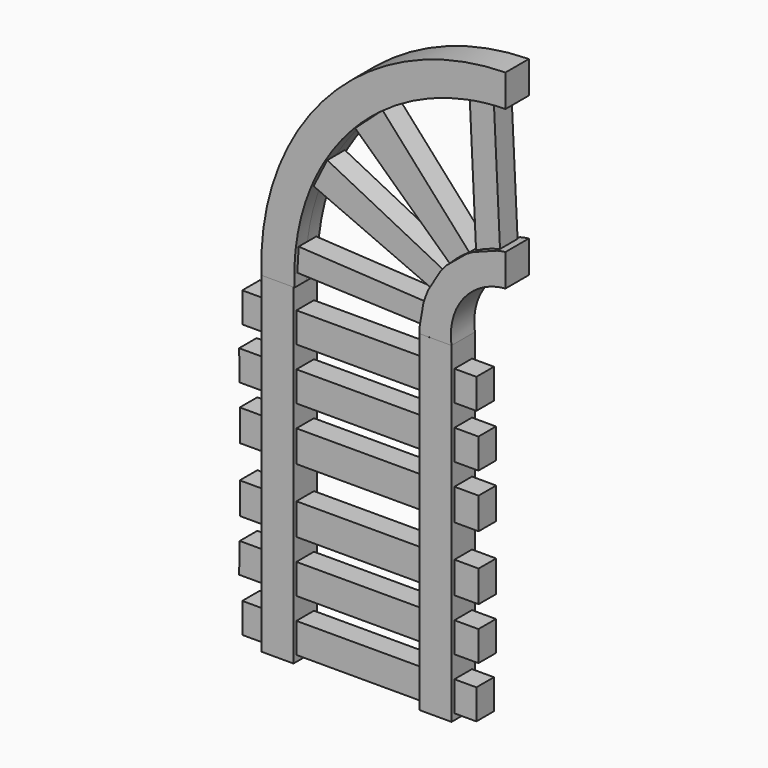
from build123d import *

# Parameters (mm, degrees)
F0_W          = 11.176
F0_H          = 7.62
F0_H_2        = 10.414
F0_H_3        = 10.414198041
F0_H_4        = 10.8981402591
F0_H_5        = 11.3893379234
F0_H_6        = 2.1167141254
F1_DEPTH      = 5.08
F1_DEPTH_BACK = 5.08
F0_W_2        = 43.688
F0_W_3        = 7.62
F0_W_4        = 8.491490941
F0_W_5        = 8.3875925946
F0_W_6        = 8.3293178785
F2_DEPTH      = 3.81
F2_DEPTH_BACK = 3.81
F4_DEPTH      = 5.08
F4_DEPTH_BACK = 5.08
F5_DEPTH      = 3.81
F5_DEPTH_BACK = 3.81


# Not quite as in the source:
# - a feature names something its author has since deleted; it is built from what else it names


with BuildPart() as f1:
    # F0 (on Front) → F1 (new body, two sides)
    with BuildSketch(Plane.XZ) as f1_sk:
        with Locations((-27.432, 56.4710072617)):
            Rectangle(F0_W, F0_H)
        with Locations((-27.432, 47.4540072617)):
            Rectangle(F0_W, F0_H_2)
        with Locations((-27.432, 38.4370072617)):
            Rectangle(F0_W, F0_H)
        with Locations((-27.432, 29.4199082413)):
            Rectangle(F0_W, F0_H_3)
        with Locations((-27.432, 20.4028092208)):
            Rectangle(F0_W, F0_H)
        with Locations((-27.432, 11.1437390912)):
            Rectangle(F0_W, F0_H_4)
        with Locations((-27.432, 0)):
            Rectangle(F0_W, F0_H_5)
        with Locations((-27.432, -11.1437390912)):
            Rectangle(F0_W, F0_H_4)
        with Locations((-27.432, -20.4028092208)):
            Rectangle(F0_W, F0_H)
        with Locations((-27.432, -29.4199082413)):
            Rectangle(F0_W, F0_H_3)
        with Locations((-27.432, -38.4370072617)):
            Rectangle(F0_W, F0_H)
        with Locations((-27.432, -47.4540072617)):
            Rectangle(F0_W, F0_H_2)
        with Locations((-27.432, -53.7193643245)):
            Rectangle(F0_W, F0_H_6)
    extrude(amount=F1_DEPTH)
    extrude(f1_sk.sketch, amount=-F1_DEPTH_BACK)



with BuildPart() as f1b:
    # F0 (on Front) → F1, piece 2 (new body, two sides)
    with BuildSketch(Plane.XZ) as f1_2_sk:
        with Locations((27.432, -47.4540072617)):
            Rectangle(F0_W, F0_H_2)
        with Locations((27.432, -38.4370072617)):
            Rectangle(F0_W, F0_H)
        with Locations((27.432, -29.4199082413)):
            Rectangle(F0_W, F0_H_3)
        with Locations((27.432, -20.4028092208)):
            Rectangle(F0_W, F0_H)
        with Locations((27.432, -11.1437390912)):
            Rectangle(F0_W, F0_H_4)
        with Locations((27.432, 0)):
            Rectangle(F0_W, F0_H_5)
        with Locations((27.432, 11.1437390912)):
            Rectangle(F0_W, F0_H_4)
        with Locations((27.432, 20.4028092208)):
            Rectangle(F0_W, F0_H)
        with Locations((27.432, 29.4199082413)):
            Rectangle(F0_W, F0_H_3)
        with Locations((27.432, 38.4370072617)):
            Rectangle(F0_W, F0_H)
        with Locations((27.432, 47.4540072617)):
            Rectangle(F0_W, F0_H_2)
        with Locations((27.432, 56.4710072617)):
            Rectangle(F0_W, F0_H)
        with Locations((27.432, -53.7193643245)):
            Rectangle(F0_W, F0_H_6)
    extrude(amount=F1_DEPTH)
    extrude(f1_2_sk.sketch, amount=-F1_DEPTH_BACK)


with BuildPart() as f1_1:
    add(f1.part)

    add(f1b.part)  # F2 merges F1b
    # F0 (on Front) → F2 (join, two sides)
    with BuildSketch(Plane.XZ) as f2_sk:
        with Locations((0, 29.4199082413)):
            Rectangle(F0_W_2, F0_H_3)
        with Locations((0, 47.4540072617)):
            Rectangle(F0_W_2, F0_H_2)
        with Locations((-36.83, 47.4540072617)):
            Rectangle(F0_W_3, F0_H_2)
        Polygon((-33.02, 24.2128092208), (-33.02, 34.6270072617), (-41.7378880084, 34.6270072617), (-41.511490941, 24.2128092208), align=None)
        with Locations((-37.2657454705, 11.1437390912)):
            Rectangle(F0_W_4, F0_H_4)
        with Locations((-37.2657454705, -11.1437390912)):
            Rectangle(F0_W_4, F0_H_4)
        with Locations((0, -11.1437390912)):
            Rectangle(F0_W_2, F0_H_4)
        with Locations((0, 11.1437390912)):
            Rectangle(F0_W_2, F0_H_4)
        with Locations((37.2137962973, -11.1437390912)):
            Rectangle(F0_W_5, F0_H_4)
        with Locations((37.2137962973, 11.1437390912)):
            Rectangle(F0_W_5, F0_H_4)
        with Locations((37.1846589392, 29.4199082413)):
            Rectangle(F0_W_6, F0_H_3)
        with Locations((36.83, 47.4540072617)):
            Rectangle(F0_W_3, F0_H_2)
        with Locations((37.1846589392, -29.4199082413)):
            Rectangle(F0_W_6, F0_H_3)
        with Locations((36.83, -47.4540072617)):
            Rectangle(F0_W_3, F0_H_2)
        with Locations((0, -47.4540072617)):
            Rectangle(F0_W_2, F0_H_2)
        with Locations((0, -29.4199082413)):
            Rectangle(F0_W_2, F0_H_3)
        Polygon((-33.02, -34.6270072617), (-33.02, -24.2128092208), (-41.511490941, -24.2128092208), (-41.7378880084, -34.6270072617), align=None)
        with Locations((-36.83, -47.4540072617)):
            Rectangle(F0_W_3, F0_H_2)
    extrude(amount=F2_DEPTH)
    extrude(f2_sk.sketch, amount=-F2_DEPTH_BACK)


with BuildPart() as f4:
    # F3 (on Front) → F4 (new body, two sides)
    with BuildSketch(Plane.XZ) as f4_sk:
        with BuildLine():
            ThreePointArc((46.7234483179, 138.3806666389), (49.2422027189, 138.5530795685), (51.7653487623, 138.6401657047))
            Line((51.7653487623, 138.6401657047), (51.7653487623, 149.8161657047))
            ThreePointArc((51.7653487623, 149.8161657047), (-9.4395332477, 122.8806362111), (-32.9566933215, 60.2826848626))
            Line((-32.9566933215, 60.2826848626), (-21.428527605, 60.2815099882))
            ThreePointArc((-21.428527605, 60.2815099882), (-21.5025853928, 62.2708854301), (-21.523534037, 64.2615286325))
            ThreePointArc((-21.523534037, 64.2615286325), (-21.4006641675, 68.3361772977), (-21.0554041735, 72.3980308506))
            ThreePointArc((-21.0554041735, 72.3980308506), (-19.1641769465, 82.6655299595), (-15.8580723991, 92.56845635))
            ThreePointArc((-15.8580723991, 92.56845635), (-13.6603359913, 97.3889321711), (-11.1260263684, 102.0412764398))
            ThreePointArc((-11.1260263684, 102.0412764398), (-6.6341482531, 108.7708829528), (-1.4398843374, 114.9744460578))
            ThreePointArc((-1.4398843374, 114.9744460578), (3.1297417642, 119.4636171712), (8.0676414189, 123.5442160236))
            ThreePointArc((8.0676414189, 123.5442160236), (22.4302043573, 132.0660955879), (38.328636759, 137.1793619255))
            ThreePointArc((38.328636759, 137.1793619255), (42.5089587111, 137.8993974077), (46.7234483179, 138.3806666389))
        make_face()
    extrude(amount=F4_DEPTH)
    extrude(f4_sk.sketch, amount=-F4_DEPTH_BACK)



with BuildPart() as f4b:
    # F3 (on Front) → F4, piece 2 (new body, two sides)
    with BuildSketch(Plane.XZ) as f4_2_sk:
        with BuildLine():
            ThreePointArc((33.0161936581, 60.2826066315), (37.2635168322, 76.1212177757), (51.7653487623, 83.7761657047))
            Line((51.7653487623, 83.7761657047), (51.7653487623, 94.9521657047))
            ThreePointArc((51.7653487623, 94.9521657047), (50.2978144115, 94.7028376295), (48.8422158841, 94.3913019379))
            Line((48.8422158841, 94.3913019379), (40.539710538, 91.2735568742))
            ThreePointArc((40.539710538, 91.2735568742), (39.3520349882, 90.6158567529), (38.190774115, 89.9125674487))
            Line((38.190774115, 89.9125674487), (31.4069914905, 84.3135852358))
            ThreePointArc((31.4069914905, 84.3135852358), (30.2440044025, 83.0135126621), (29.1472703966, 81.6570827214))
            Line((29.1472703966, 81.6570827214), (24.9918396341, 74.709399156))
            ThreePointArc((24.9918396341, 74.709399156), (24.0278925704, 72.340750689), (23.2395618841, 69.9080106226))
            Line((23.2395618841, 69.9080106226), (21.9797545722, 62.5895138801))
            ThreePointArc((21.9797545722, 62.5895138801), (21.9248040705, 61.4366528948), (21.9079152744, 60.2826066315))
            Line((21.9079152744, 60.2826066315), (33.0161936581, 60.2826066315))
        make_face()
    extrude(amount=F4_DEPTH)
    extrude(f4_2_sk.sketch, amount=-F4_DEPTH_BACK)


with BuildPart() as f4_1:
    add(f4.part)

    add(f4b.part)  # F5 merges F4b
    # F3 (on Front) → F5 (join, two sides)
    with BuildSketch(Plane.XZ) as f5_sk:
        with BuildLine():
            Line((-21.523534037, 64.2615286325), (21.9797545722, 62.5895138801))
            ThreePointArc((21.9797545722, 62.5895138801), (22.4149059417, 66.2822869441), (23.2395618841, 69.9080106226))
            Line((23.2395618841, 69.9080106226), (-21.0554041735, 72.3980308506))
            Line((-21.0554041735, 72.3980308506), (-21.523534037, 64.2615286325))
        make_face()
        with BuildLine():
            Line((-15.8580723991, 92.56845635), (24.9918396341, 74.709399156))
            ThreePointArc((24.9918396341, 74.709399156), (26.8678964449, 78.3038535456), (29.1472703966, 81.6570827214))
            Line((29.1472703966, 81.6570827214), (-11.1260263684, 102.0412764398))
            Line((-11.1260263684, 102.0412764398), (-15.8580723991, 92.56845635))
        make_face()
        with BuildLine():
            ThreePointArc((31.4069914905, 84.3135852358), (34.6222032412, 87.327143059), (38.190774115, 89.9125674487))
            Line((38.190774115, 89.9125674487), (8.0676414189, 123.5442160236))
            Line((8.0676414189, 123.5442160236), (-1.4398843374, 114.9744460578))
            Line((-1.4398843374, 114.9744460578), (31.4069914905, 84.3135852358))
        make_face()
        with BuildLine():
            ThreePointArc((40.539710538, 91.2735568742), (44.5917613588, 93.0966023555), (48.8422158841, 94.3913019379))
            Line((48.8422158841, 94.3913019379), (46.7234483179, 138.3806666389))
            Line((46.7234483179, 138.3806666389), (38.328636759, 137.1793619255))
            Line((38.328636759, 137.1793619255), (40.539710538, 91.2735568742))
        make_face()
    extrude(amount=F5_DEPTH)
    extrude(f5_sk.sketch, amount=-F5_DEPTH_BACK)


solid = Compound([f1_1.part, f4_1.part])
